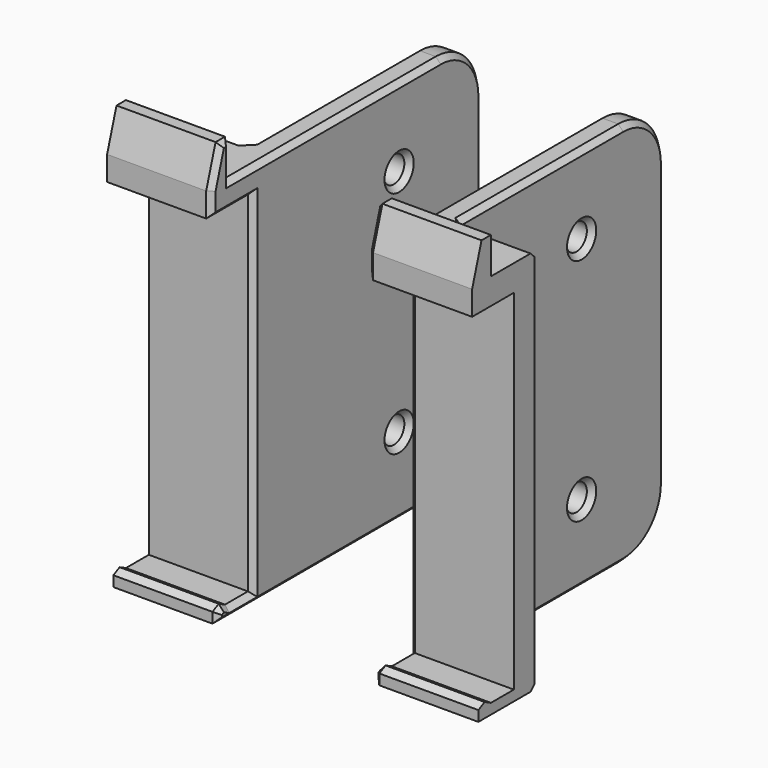
from build123d import *

# Parameters (mm, degrees)
F1_DEPTH = 10
F2_W     = 5
F2_H     = 74
F3_DEPTH = 50
F4_R     = 2.5
F5_DEPTH = 5
F6_R     = 10
F7_SIZE  = 0.99999


# Not quite as in the source:
# - a fillet or chamfer is up to 0.001 mm smaller than in the source, because OpenCascade refuses the exact size


with BuildPart() as f1:
    # F0 (on Right) → F1 (new body, symmetric)
    with BuildSketch(Plane.YZ):
        Polygon((-23.9496866415, 58.3136815727), (-23.9496866415, -8.6863184273), (-29.4496866415, -8.6863184273), (-30.9496866415, -7.9363184273), (-32.4496866415, -8.6863184273), (-32.4496866415, -10.6863184273), (-18.9496866415, -10.6863184273), (-18.9496866415, 63.3136815727), (-29.4496866415, 63.3136815727), (-29.4496866415, 70.3136815727), (-31.6996866415, 70.3136815727), (-33.9496866415, 62.9810988903), (-33.9496866415, 58.3136815727), align=None)
    extrude(amount=F1_DEPTH, both=True)

    # F2 (on face) → F3 (join)
    with BuildSketch(Plane(origin=(0, -18.9496866415, 0), x_dir=(-1, 0, 0), z_dir=(0, 1, 0))):
        with Locations((-7.5, 26.3136815727)):
            Rectangle(F2_W, F2_H)
    extrude(amount=F3_DEPTH)

    # F4 (on face) → F5 (cut, through all)
    with BuildSketch(Plane.YZ.offset(10)):
        with Locations((11.0503133585, 48.3136815727)):
            Circle(F4_R)
        with Locations((11.0503133585, 4.3136815727)):
            Circle(F4_R)
    extrude(amount=-F5_DEPTH, mode=Mode.SUBTRACT)

    # F6
    f6_edges = [f1.edges().sort_by_distance(p)[0] for p in [
        (7.5, 31.050313, 63.313682),
        (7.5, 31.050313, -10.686318),
    ]]
    fillet(f6_edges, radius=F6_R)

    # F7 (size 1 in the source; OpenCascade refuses exactly that, so slightly less here)
    f7_edges = [f1.edges().sort_by_distance(p)[0] for p in [
        (10, -4.199687, 63.313682),
        (10, 28.121381, 60.384749),
        (10, -29.449687, 66.813682),
        (10, 31.050313, 26.313682),
        (10, -30.574687, 70.313682),
        (10, 28.121381, -7.757386),
        (10, -32.824687, 66.64739),
        (10, -5.699687, -10.686318),
        (10, -33.949687, 60.64739),
        (10, -32.449687, -9.686318),
        (10, -28.949687, 58.313682),
        (10, -31.699687, -8.311318),
        (10, -23.949687, 24.813682),
        (10, -30.199687, -8.311318),
        (10, -26.699687, -8.686318),
        (10, 8.550313, 4.313682),
        (10, 8.550313, 48.313682),
        (5, 1.050313, -10.686318),
        (5, 28.121381, -7.757386),
        (5, -18.949687, 26.313682),
        (5, 31.050313, 26.313682),
        (5, 1.050313, 63.313682),
        (5, 28.121381, 60.384749),
        (5, 8.550313, 4.313682),
        (5, 8.550313, 48.313682),
        (-2.5, -18.949687, 63.313682),
        (-2.5, -18.949687, -10.686318),
    ]]
    chamfer(f7_edges, length=F7_SIZE)


with BuildPart() as f9_1:
    # F9: instance of F1
    add(f1.part.mirror(Plane.YZ.offset(25)))


solid = Compound([f1.part, f9_1.part])
